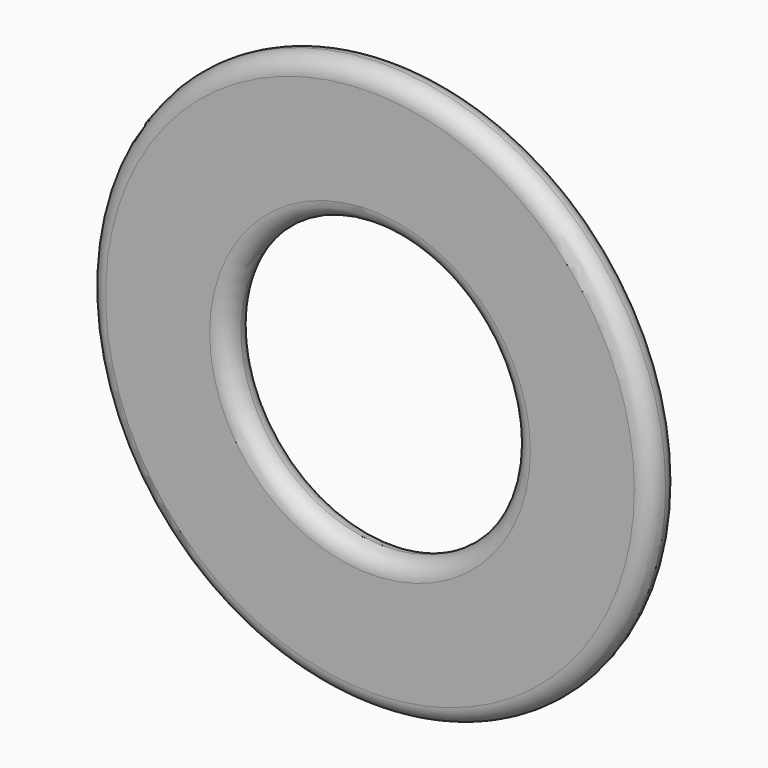
from build123d import *

# Parameters (mm, degrees)
F0_R     = 32.5
F0_R_2   = 16.5
F1_DEPTH = 4
F2_R     = 1.99999


# Not quite as in the source:
# - a fillet or chamfer is up to 0.001 mm smaller than in the source, because OpenCascade refuses the exact size
# - a feature names something its author has since deleted; it is built from what else it names


with BuildPart() as f1:
    # F0 (on Front) → F1 (new body)
    with BuildSketch(Plane.XZ):
        Circle(F0_R)
        Circle(F0_R_2, mode=Mode.SUBTRACT)
    extrude(amount=F1_DEPTH)

    # F2 (radius 2 in the source; OpenCascade refuses exactly that, so slightly less here)
    f2_edges = [f1.edges().sort_by_distance(p)[0] for p in [
        (-32.5, -4, 0),
        (-32.5, 0, 0),
        (-16.5, 0, 0),
        (-16.5, -4, 0),
    ]]
    fillet(f2_edges, radius=F2_R)


solid = f1.part
